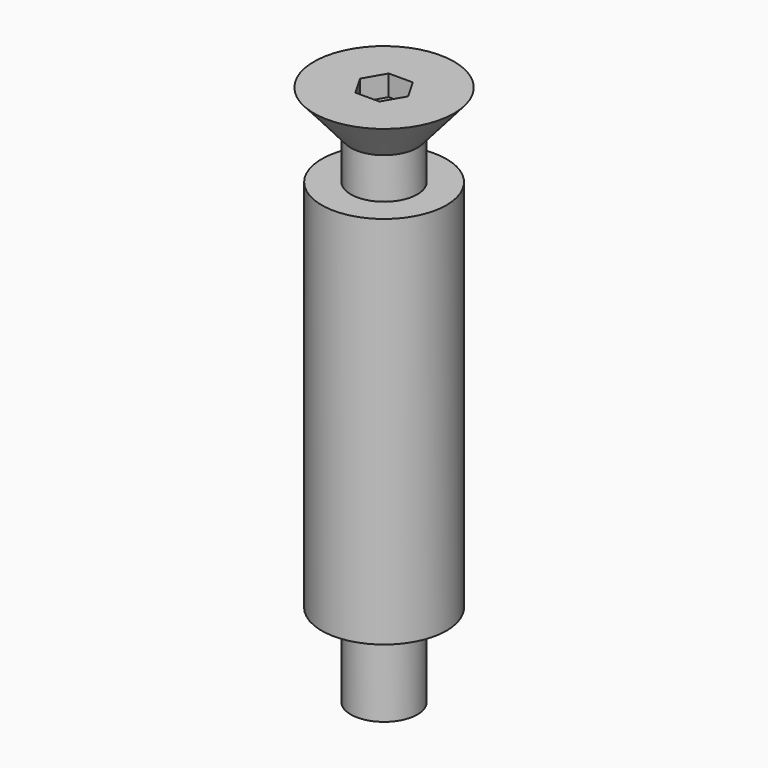
from build123d import *

# Parameters (mm, degrees)
F3_DEPTH = 1.5875


with BuildPart() as f1:
    # F0 (on Front) → F1 (revolve)
    with BuildSketch(Plane.XZ):
        Polygon((5.3441451588, 0), (0, 0), (0, -3.2258), (0, -41.275), (2.54, -41.275), (2.54, -34.925), (4.7625, -34.925), (4.7625, -6.35), (2.54, -6.35), (2.54, -3.2258), align=None)
    revolve(axis=Axis((0, 0, -22.2504), (0, 0, -1)))

    # F2 (on face) → F3 (cut)
    with BuildSketch(Plane.XY):
        Polygon((0.9165435523, 1.5875), (-0.9165435523, 1.5875), (-1.8330871047, 0), (-0.9165435523, -1.5875), (0.9165435523, -1.5875), (1.8330871047, 0), align=None)
    extrude(amount=-F3_DEPTH, mode=Mode.SUBTRACT)


solid = f1.part
